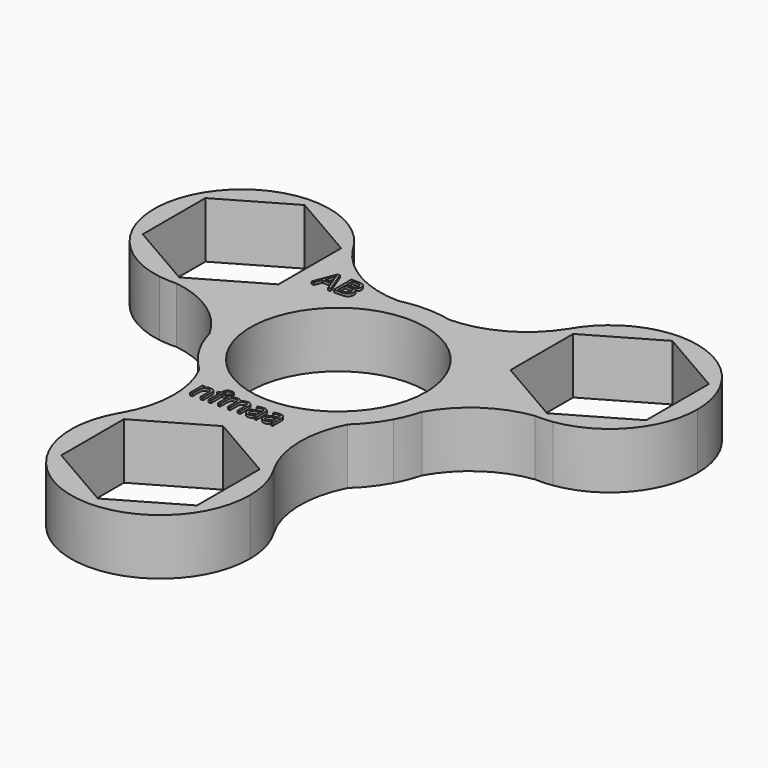
from build123d import *

# Parameters (mm, degrees)
F0_R           = 10.9719272867
F1_DEPTH       = 7
F2_TEXT_SIZE   = 3.6541450148
F2_TEXT_SIZE_2 = 3.8281509963
F3_DEPTH       = 7.3


# Not quite as in the source:
# - Text() gives the source's letters only with a copy of the font that has no kerning and outlines rounded to 1/6400 em; it was checked with that copy


with BuildPart() as f1:
    # F0 (on Top) → F1 (new body)
    with BuildSketch(Plane.XY):
        with BuildLine():
            ThreePointArc((13.2711358157, -3.5440166875), (13.6194352357, -1.7872000391), (13.7361967123, 0))
            ThreePointArc((13.7361967123, 0), (10.7714308236, 8.5240470513), (3.1569396364, 13.3685014961))
            ThreePointArc((3.1569396364, 13.3685014961), (1.5666454361, 13.4508279018), (0, 13.7361967123))
            ThreePointArc((0, 13.7361967123), (-1.5666454361, 13.4508279018), (-3.1569396364, 13.3685014961))
            ThreePointArc((-3.1569396364, 13.3685014961), (-11.7889241915, 7.0501323766), (-13.2711358157, -3.5440166875))
            ThreePointArc((-13.2711358157, -3.5440166875), (-12.584121889, -4.993925787), (-12.0899866465, -6.5203775204))
            ThreePointArc((-12.0899866465, -6.5203775204), (-10.5155940661, -8.1944331859), (-9.2770038263, -10.1301678232))
            ThreePointArc((-9.2770038263, -10.1301678232), (0, -13.7361967123), (9.2770038263, -10.1301678232))
            ThreePointArc((9.2770038263, -10.1301678232), (10.5155940661, -8.1944331859), (12.0899866465, -6.5203775204))
            ThreePointArc((12.0899866465, -6.5203775204), (12.584121889, -4.993925787), (13.2711358157, -3.5440166875))
        make_face()
        Circle(F0_R, mode=Mode.SUBTRACT)
        with BuildLine():
            ThreePointArc((3.1569396364, 13.3685014961), (10.7714308236, 8.5240470513), (13.7361967123, 0))
            ThreePointArc((13.7361967123, 0), (13.6194352357, -1.7872000391), (13.2711358157, -3.5440166875))
            ThreePointArc((13.2711358157, -3.5440166875), (17.1067253124, 0.6664640874), (22.4195716771, 2.7191595464))
            ThreePointArc((22.4195716771, 2.7191595464), (13.3804416715, 8.387709783), (13.4320212737, 19.0570899237))
            ThreePointArc((13.4320212737, 19.0570899237), (9.0103342367, 14.9197761602), (3.1569396364, 13.3685014961))
        make_face()
        with BuildLine():
            ThreePointArc((0, 13.7361967123), (1.5666454361, 13.4508279018), (3.1569396364, 13.3685014961))
            ThreePointArc((3.1569396364, 13.3685014961), (1.5891403053, 13.6439632516), (0, 13.7361967123))
        make_face()
        with BuildLine():
            ThreePointArc((12.0899866465, -6.5203775204), (12.767588421, -5.0667332704), (13.2711358157, -3.5440166875))
            ThreePointArc((13.2711358157, -3.5440166875), (12.584121889, -4.993925787), (12.0899866465, -6.5203775204))
        make_face()
        with BuildLine():
            ThreePointArc((-3.1569396364, 13.3685014961), (-1.5666454361, 13.4508279018), (0, 13.7361967123))
            ThreePointArc((0, 13.7361967123), (-1.5891403053, 13.6439632516), (-3.1569396364, 13.3685014961))
        make_face()
        with BuildLine():
            ThreePointArc((33.9657265857, 13.6760501191), (25.7751708275, 24.2895867966), (13.4320212737, 19.0570899237))
            ThreePointArc((13.4320212737, 19.0570899237), (13.3804416715, 8.387709783), (22.4195716771, 2.7191595464))
            ThreePointArc((22.4195716771, 2.7191595464), (23.5171682341, 2.8211127186), (24.6194820356, 2.825227845))
            ThreePointArc((24.6194820356, 2.825227845), (31.3070435864, 6.515522359), (33.9657265857, 13.6760501191))
        make_face()
        Polygon((22.993799299, 23.4742843433), (31.4793190494, 18.5751672312), (31.4793190494, 8.776933007), (22.993799299, 3.8778158949), (14.5082795486, 8.776933007), (14.5082795486, 18.5751672312), align=None, mode=Mode.SUBTRACT)
        with BuildLine():
            ThreePointArc((9.2770038263, -10.1301678232), (10.8348842621, -8.4432448233), (12.0899866465, -6.5203775204))
            ThreePointArc((12.0899866465, -6.5203775204), (10.5155940661, -8.1944331859), (9.2770038263, -10.1301678232))
        make_face()
        with BuildLine():
            ThreePointArc((24.6194820356, 2.825227845), (23.5171682341, 2.8211127186), (22.4195716771, 2.7191595464))
            ThreePointArc((22.4195716771, 2.7191595464), (23.522195065, 2.7168536933), (24.6194820356, 2.825227845))
        make_face()
        with BuildLine():
            ThreePointArc((-13.2711358157, -3.5440166875), (-11.7889241915, 7.0501323766), (-3.1569396364, 13.3685014961))
            ThreePointArc((-3.1569396364, 13.3685014961), (-9.0103342367, 14.9197761602), (-13.4320212737, 19.0570899237))
            ThreePointArc((-13.4320212737, 19.0570899237), (-12.3802626215, 16.4574216476), (-12.0218720123, 13.6760501191))
            ThreePointArc((-12.0218720123, 13.6760501191), (-15.0350439912, 6.1234742449), (-22.4195716771, 2.7191595464))
            ThreePointArc((-22.4195716771, 2.7191595464), (-17.1067253124, 0.6664640874), (-13.2711358157, -3.5440166875))
        make_face()
        with BuildLine():
            ThreePointArc((9.5333938521, -21.9804282169), (7.8983078809, -16.0879008321), (9.2770038263, -10.1301678232))
            ThreePointArc((9.2770038263, -10.1301678232), (0, -13.7361967123), (-9.2770038263, -10.1301678232))
            ThreePointArc((-9.2770038263, -10.1301678232), (-7.8983078809, -16.0879008321), (-9.5333938521, -21.9804282169))
            ThreePointArc((-9.5333938521, -21.9804282169), (0, -16.6321272459), (9.5333938521, -21.9804282169))
        make_face()
        with BuildLine():
            ThreePointArc((-12.0899866465, -6.5203775204), (-12.584121889, -4.993925787), (-13.2711358157, -3.5440166875))
            ThreePointArc((-13.2711358157, -3.5440166875), (-12.767588421, -5.0667332704), (-12.0899866465, -6.5203775204))
        make_face()
        with BuildLine():
            ThreePointArc((-12.0218720123, 13.6760501191), (-12.3802626215, 16.4574216476), (-13.4320212737, 19.0570899237))
            ThreePointArc((-13.4320212737, 19.0570899237), (-32.0278315518, 19.9025619549), (-24.6194820356, 2.825227845))
            ThreePointArc((-24.6194820356, 2.825227845), (-23.5171682341, 2.8211127186), (-22.4195716771, 2.7191595464))
            ThreePointArc((-22.4195716771, 2.7191595464), (-15.0350439912, 6.1234742449), (-12.0218720123, 13.6760501191))
        make_face()
        Polygon((-22.993799299, 23.4742843433), (-14.5082795486, 18.5751672312), (-14.5082795486, 8.776933007), (-22.993799299, 3.8778158949), (-31.4793190494, 8.776933007), (-31.4793190494, 18.5751672312), align=None, mode=Mode.SUBTRACT)
        with BuildLine():
            ThreePointArc((-12.0899866465, -6.5203775204), (-10.8348842621, -8.4432448233), (-9.2770038263, -10.1301678232))
            ThreePointArc((-9.2770038263, -10.1301678232), (-10.5155940661, -8.1944331859), (-12.0899866465, -6.5203775204))
        make_face()
        with BuildLine():
            ThreePointArc((9.7041195554, -22.2696484463), (9.6177778899, -22.125616122), (9.5333938521, -21.9804282169))
            ThreePointArc((9.5333938521, -21.9804282169), (0, -16.6321272459), (-9.5333938521, -21.9804282169))
            ThreePointArc((-9.5333938521, -21.9804282169), (-9.6177778899, -22.125616122), (-9.7041195554, -22.2696484463))
            ThreePointArc((-9.7041195554, -22.2696484463), (-2.8621995678, -38.600885541), (11.170829976, -27.8029572219))
            ThreePointArc((11.170829976, -27.8029572219), (10.7979283192, -24.9407576541), (9.7041195554, -22.2696484463))
        make_face()
        Polygon((0, -18.0047229977), (8.4855197504, -22.9038401098), (8.4855197504, -32.7020743339), (0, -37.601191446), (-8.4855197504, -32.7020743339), (-8.4855197504, -22.9038401098), align=None, mode=Mode.SUBTRACT)
        with BuildLine():
            ThreePointArc((9.7041195554, -22.2696484463), (9.6198436895, -22.1243966876), (9.5333938521, -21.9804282169))
            ThreePointArc((9.5333938521, -21.9804282169), (9.6177778899, -22.125616122), (9.7041195554, -22.2696484463))
        make_face()
        with BuildLine():
            ThreePointArc((-24.6194820356, 2.825227845), (-23.522195065, 2.7168536933), (-22.4195716771, 2.7191595464))
            ThreePointArc((-22.4195716771, 2.7191595464), (-23.5171682341, 2.8211127186), (-24.6194820356, 2.825227845))
        make_face()
        with BuildLine():
            ThreePointArc((-9.7041195554, -22.2696484463), (-9.6177778899, -22.125616122), (-9.5333938521, -21.9804282169))
            ThreePointArc((-9.5333938521, -21.9804282169), (-9.6198436895, -22.1243966876), (-9.7041195554, -22.2696484463))
        make_face()
    extrude(amount=F1_DEPTH)

    # F2 (on Top) → F3 (join)
    with BuildSketch(Plane.XY):
        with Locations((-6.8894140422, -14.9661870673)):
            Text('nfmaa', F2_TEXT_SIZE, font='Open Sans', text_align=(TextAlign.LEFT, TextAlign.BOTTOM))
        with Locations((-12.0260966942, 10.8425142244)):
            Text('AB', F2_TEXT_SIZE_2, font='Open Sans', text_align=(TextAlign.LEFT, TextAlign.BOTTOM))
    extrude(amount=F3_DEPTH)


solid = f1.part
